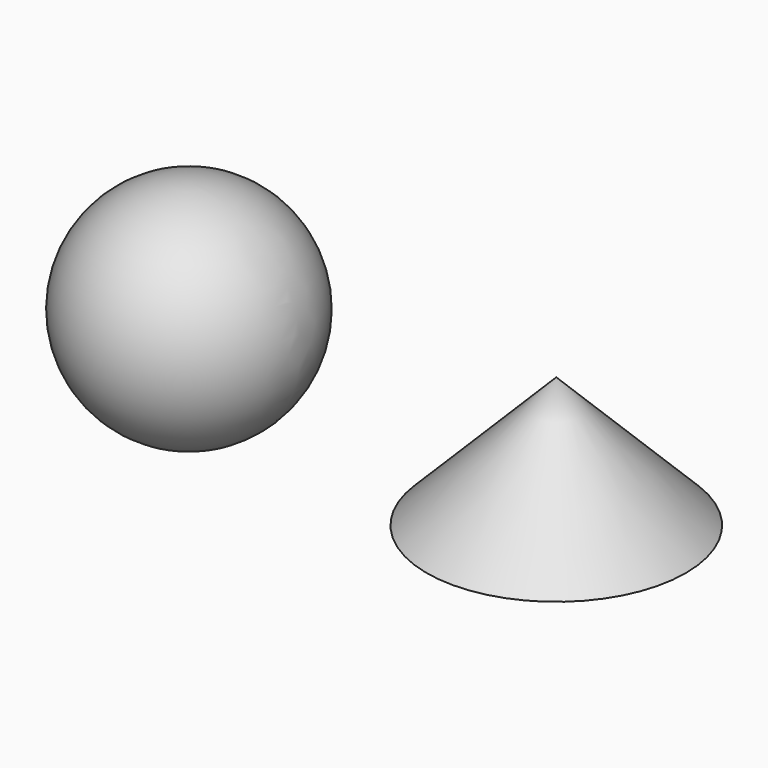
from build123d import *


with BuildPart() as f1:
    # F0 (on Front) → F1 (revolve)
    with BuildSketch(Plane.XZ):
        Polygon((-379.1255354881, 762.6939415932), (-379.1255354881, -179.1960597038), (556.8405985832, -179.1960597038), align=None)
    revolve(axis=Axis((-379.1255354881, 0, 291.7489409447), (0, 0, 1)))


with BuildPart() as f3:
    # F2 (on Front) → F3 (revolve)
    with BuildSketch(Plane.XZ):
        with BuildLine():
            ThreePointArc((-3033.9803695679, -472.5624929023), (-2463.913454472, -236.4330452094), (-2227.7840067791, 333.6338698864))
            ThreePointArc((-2227.7840067791, 333.6338698864), (-2463.913454472, 903.7007849822), (-3033.9803695679, 1139.8302326751))
            Line((-3033.9803695679, 1139.8302326751), (-3033.9803695679, 333.6338698864))
            Line((-3033.9803695679, 333.6338698864), (-3033.9803695679, -472.5624929023))
        make_face()
    revolve(axis=Axis((-3033.9803695679, 0, 333.6338698864), (0, 0, 1)))


solid = Compound([f1.part, f3.part])
